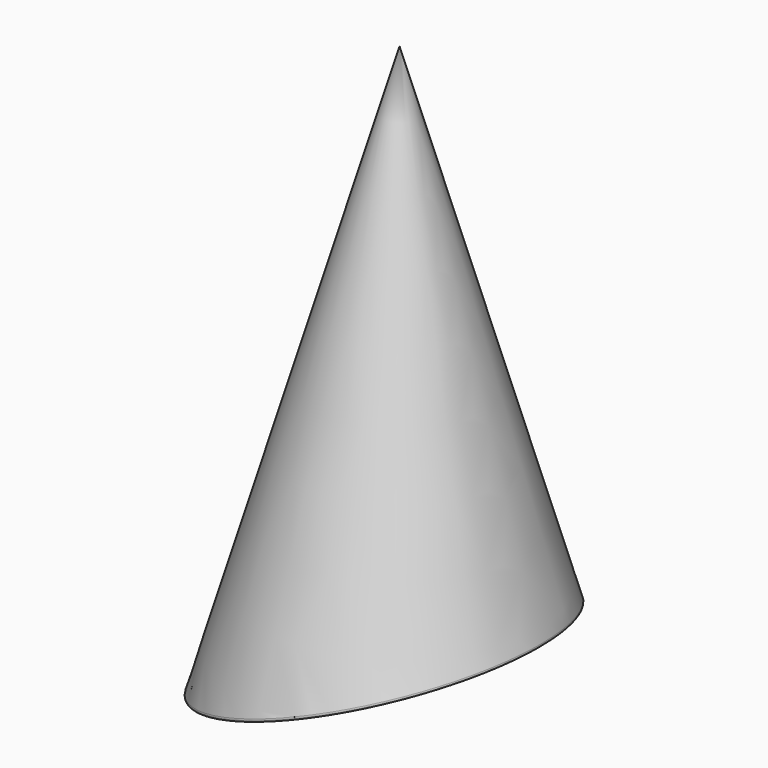
from build123d import *

# Parameters (mm, degrees)
F2_R     = 1.5
F5_DEPTH = 55.3
F6_T     = -2
F8_R     = 0.2


# Not quite as in the source:
# - a feature of the source that left no trace in its solid (it failed there, or was rolled back) is left out


with BuildPart() as f1:
    # F0 (on Front) → F1 (revolve)
    with BuildSketch(Plane.XZ):
        Polygon((0, 32.9506285489), (0, -27.0493714511), (17.5, -27.0493714511), align=None)
    revolve(axis=Axis((0, 0, 2.9506285489), (0, 0, -1)))

    # F2
    f2_edges = [f1.edges().sort_by_distance(p)[0] for p in [
        (-17.5, 0, -27.049371),
    ]]
    fillet(f2_edges, radius=F2_R)

    # F4 (on offset) → F5 (cut)
    with BuildSketch(Plane.XZ.offset(25)):
        Polygon((11.7434896529, -7.0389136672), (-14.4568033888, -16.1161629583), (-22.2343672067, -16.070589817), (-22.2343672067, -30.6586939842), (20.5961283824, -30.6586939842), (20.5961283824, -7.1517258466), align=None)
    extrude(amount=-F5_DEPTH, mode=Mode.SUBTRACT)

    # F6
    f6_openings = [f1.faces().sort_by_distance(p)[0] for p in [
        (-1.311914, 0, -11.562037),
    ]]
    offset(amount=F6_T, openings=f6_openings)

    # F8
    f8_edges = [f1.edges().sort_by_distance(p)[0] for p in [
        (-14.294775, 0, -16.060027),
        (-11.977257, 0, -15.257109),
    ]]
    fillet(f8_edges, radius=F8_R)


solid = f1.part
